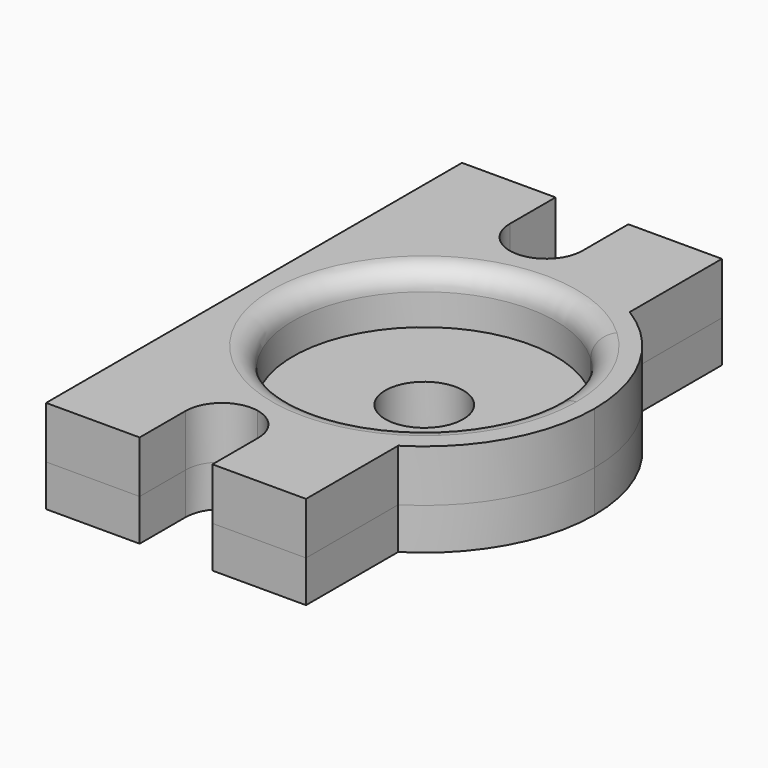
from build123d import *

# Parameters (mm, degrees)
F0_R     = 1.905
F1_DEPTH = 2.032
F2_DEPTH = 2.54
F3_R     = 1.016


# Not quite as in the source:
# - a feature names something its author has since deleted; it is built from what else it names


with BuildPart() as f1:
    # F0 (on Top) → F1 (new body)
    with BuildSketch(Plane.XY):
        with BuildLine():
            Line((6.35, 4.6835285843), (6.35, 7.0710607408))
            ThreePointArc((6.35, 7.0710607408), (3.4516559454, 8.1852117072), (0.3466541063, 8.1588637779))
            ThreePointArc((0.3466541063, 8.1588637779), (-4.4614598428, 5.2775997073), (-6.35, 1.93e-08))
            ThreePointArc((-6.35, 1.93e-08), (-4.4614598575, -5.2775996893), (0.3466540985, -8.1588637764))
            ThreePointArc((0.3466540985, -8.1588637764), (3.4516559415, -8.1852117079), (6.35, -7.0710607408))
            Line((6.35, -7.0710607408), (6.35, -4.6835285843))
            ThreePointArc((6.35, -4.6835285843), (-4.445, 0), (6.35, 4.6835285843))
        make_face()
        with BuildLine():
            ThreePointArc((10.287, 0), (9.2364071953, 4.0465994675), (6.35, 7.0710607408))
            Line((6.35, 7.0710607408), (6.35, 4.6835285843))
            ThreePointArc((6.35, 4.6835285843), (7.8521099675, 2.5526684078), (8.382, 0))
            ThreePointArc((8.382, 0), (7.8521099675, -2.5526684078), (6.35, -4.6835285843))
            Line((6.35, -4.6835285843), (6.35, -7.0710607408))
            ThreePointArc((6.35, -7.0710607408), (9.2364071953, -4.0465994675), (10.287, 0))
        make_face()
        with BuildLine():
            Line((-1.778, 9.9027430543), (-1.778, 12.7))
            Line((-1.778, 12.7), (-6.35, 12.7))
            Line((-6.35, 12.7), (-6.35, 1.93e-08))
            ThreePointArc((-6.35, 1.93e-08), (-4.4614598428, 5.2775997073), (0.3466541063, 8.1588637779))
            ThreePointArc((0.3466541063, 8.1588637779), (-1.1280365683, 8.528400484), (-1.778, 9.9027430543))
        make_face()
        with BuildLine():
            Line((6.35, 7.0710607408), (6.35, 12.7))
            Line((6.35, 12.7), (1.778, 12.7))
            Line((1.778, 12.7), (1.778, 9.9027430543))
            ThreePointArc((1.778, 9.9027430543), (1.3743425703, 8.774706486), (0.3466541063, 8.1588637779))
            ThreePointArc((0.3466541063, 8.1588637779), (3.4516559454, 8.1852117072), (6.35, 7.0710607408))
        make_face()
        with BuildLine():
            Line((6.35, -12.7), (6.35, -7.0710607408))
            ThreePointArc((6.35, -7.0710607408), (3.4516559415, -8.1852117079), (0.3466540985, -8.1588637764))
            ThreePointArc((0.3466540985, -8.1588637764), (1.3743425678, -8.7747064829), (1.778, -9.9027430543))
            Line((1.778, -9.9027430543), (1.778, -12.7))
            Line((1.778, -12.7), (6.35, -12.7))
        make_face()
        with BuildLine():
            ThreePointArc((0.3466540985, -8.1588637764), (-4.4614598575, -5.2775996893), (-6.35, 1.93e-08))
            Line((-6.35, 1.93e-08), (-6.35, -12.7))
            Line((-6.35, -12.7), (-1.778, -12.7))
            Line((-1.778, -12.7), (-1.778, -9.9027430543))
            ThreePointArc((-1.778, -9.9027430543), (-1.1280365714, -8.5284004866), (0.3466540985, -8.1588637764))
        make_face()
        with BuildLine():
            Line((6.35, -4.6835285843), (6.35, 4.6835285843))
            ThreePointArc((6.35, 4.6835285843), (-4.445, 0), (6.35, -4.6835285843))
        make_face()
        with Locations((1.9685, 0)):
            Circle(F0_R, mode=Mode.SUBTRACT)
        with BuildLine():
            ThreePointArc((8.382, 0), (7.8521099675, 2.5526684078), (6.35, 4.6835285843))
            Line((6.35, 4.6835285843), (6.35, -4.6835285843))
            ThreePointArc((6.35, -4.6835285843), (7.8521099675, -2.5526684078), (8.382, 0))
        make_face()
    extrude(amount=-F1_DEPTH)

    # F0 (on Top) → F2 (join)
    with BuildSketch(Plane.XY):
        with BuildLine():
            Line((6.35, 4.6835285843), (6.35, 7.0710607408))
            ThreePointArc((6.35, 7.0710607408), (3.4516559454, 8.1852117072), (0.3466541063, 8.1588637779))
            ThreePointArc((0.3466541063, 8.1588637779), (-4.4614598428, 5.2775997073), (-6.35, 1.93e-08))
            ThreePointArc((-6.35, 1.93e-08), (-4.4614598575, -5.2775996893), (0.3466540985, -8.1588637764))
            ThreePointArc((0.3466540985, -8.1588637764), (3.4516559415, -8.1852117079), (6.35, -7.0710607408))
            Line((6.35, -7.0710607408), (6.35, -4.6835285843))
            ThreePointArc((6.35, -4.6835285843), (-4.445, 0), (6.35, 4.6835285843))
        make_face()
        with BuildLine():
            ThreePointArc((10.287, 0), (9.2364071953, 4.0465994675), (6.35, 7.0710607408))
            Line((6.35, 7.0710607408), (6.35, 4.6835285843))
            ThreePointArc((6.35, 4.6835285843), (7.8521099675, 2.5526684078), (8.382, 0))
            ThreePointArc((8.382, 0), (7.8521099675, -2.5526684078), (6.35, -4.6835285843))
            Line((6.35, -4.6835285843), (6.35, -7.0710607408))
            ThreePointArc((6.35, -7.0710607408), (9.2364071953, -4.0465994675), (10.287, 0))
        make_face()
        with BuildLine():
            Line((6.35, 7.0710607408), (6.35, 12.7))
            Line((6.35, 12.7), (1.778, 12.7))
            Line((1.778, 12.7), (1.778, 9.9027430543))
            ThreePointArc((1.778, 9.9027430543), (1.3743425703, 8.774706486), (0.3466541063, 8.1588637779))
            ThreePointArc((0.3466541063, 8.1588637779), (3.4516559454, 8.1852117072), (6.35, 7.0710607408))
        make_face()
        with BuildLine():
            Line((-1.778, 9.9027430543), (-1.778, 12.7))
            Line((-1.778, 12.7), (-6.35, 12.7))
            Line((-6.35, 12.7), (-6.35, 1.93e-08))
            ThreePointArc((-6.35, 1.93e-08), (-4.4614598428, 5.2775997073), (0.3466541063, 8.1588637779))
            ThreePointArc((0.3466541063, 8.1588637779), (-1.1280365683, 8.528400484), (-1.778, 9.9027430543))
        make_face()
        with BuildLine():
            Line((6.35, -12.7), (6.35, -7.0710607408))
            ThreePointArc((6.35, -7.0710607408), (3.4516559415, -8.1852117079), (0.3466540985, -8.1588637764))
            ThreePointArc((0.3466540985, -8.1588637764), (1.3743425678, -8.7747064829), (1.778, -9.9027430543))
            Line((1.778, -9.9027430543), (1.778, -12.7))
            Line((1.778, -12.7), (6.35, -12.7))
        make_face()
        with BuildLine():
            ThreePointArc((0.3466540985, -8.1588637764), (-4.4614598575, -5.2775996893), (-6.35, 1.93e-08))
            Line((-6.35, 1.93e-08), (-6.35, -12.7))
            Line((-6.35, -12.7), (-1.778, -12.7))
            Line((-1.778, -12.7), (-1.778, -9.9027430543))
            ThreePointArc((-1.778, -9.9027430543), (-1.1280365714, -8.5284004866), (0.3466540985, -8.1588637764))
        make_face()
    extrude(amount=F2_DEPTH)

    # F3
    f3_edges = [f1.edges().sort_by_distance(p)[0] for p in [
        (-2.413, -4.683529, 2.54),
    ]]
    fillet(f3_edges, radius=F3_R)


solid = f1.part
